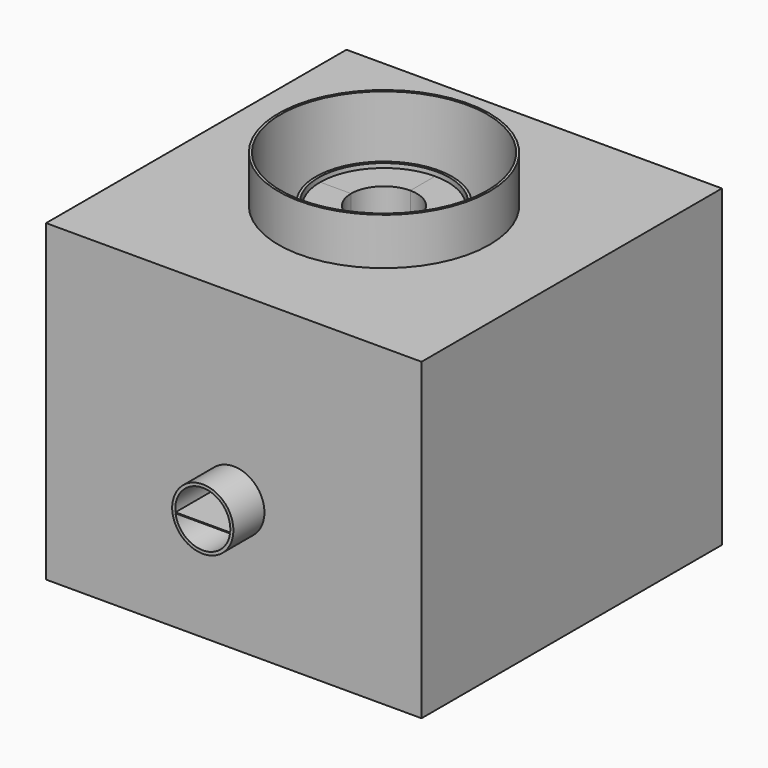
from build123d import *

# Parameters (mm, degrees)
F1_DEPTH       = 300
F0_W           = 400
F0_H           = 400
F0_R           = 112.5
F3_DEPTH       = 300
F0_R_2         = 110
F6_DEPTH       = 350
F2_W           = 400
F2_H           = 400
F7_DEPTH       = 10
F7_DEPTH_BACK  = 34.37157
F8_DEPTH       = 300
F9_R           = 72.7369791191
F9_R_2         = 69.9297965839
F10_DEPTH      = 293.61576
F4_R           = 30
F11_DEPTH      = 200.001
F12_R          = 32.6159593981
F12_R_2        = 29.3425223408
F13_DEPTH      = 41.30995
F13_DEPTH_BACK = 188.14221
F15_DEPTH      = 41.30995
F15_DEPTH_BACK = 187.07896
F16_R          = 35.0632832386
F17_DEPTH      = 410.93389


with BuildPart() as f1:
    # F0 (on Top) → F1 (new body)
    with BuildSketch(Plane.XY):
        with BuildLine():
            Line((0, 35), (0, 68))
            ThreePointArc((0, 68), (-48.0832611207, 48.0832611207), (-68, 0))
            Line((-68, 0), (-35, 0))
            ThreePointArc((-35, 0), (-24.7487373415, 24.7487373415), (0, 35))
        make_face()
    extrude(amount=F1_DEPTH)


with BuildPart() as f1b:
    # F0 (on Top) → F1, piece 2 (new body)
    with BuildSketch(Plane.XY):
        with BuildLine():
            ThreePointArc((0, -68), (48.0832611207, -48.0832611207), (68, 0))
            Line((68, 0), (35, 0))
            ThreePointArc((35, 0), (24.7487373415, -24.7487373415), (0, -35))
            Line((0, -35), (0, -68))
        make_face()
    extrude(amount=F1_DEPTH)


with BuildPart() as f3:
    # F0 (on Top) → F3 (new body)
    with BuildSketch(Plane.XY):
        Rectangle(F0_W, F0_H)
        Circle(F0_R, mode=Mode.SUBTRACT)
    extrude(amount=F3_DEPTH)

    # F2 (on Top) → F7 (join, two sides)
    with BuildSketch(Plane.XY) as f7_sk:
        Rectangle(F2_W, F2_H)
    extrude(amount=F7_DEPTH)
    extrude(f7_sk.sketch, amount=-F7_DEPTH_BACK)

    # F9 (on face) → F10 (join)
    with BuildSketch(Plane.XY.offset(10)):
        Circle(F9_R)
        Circle(F9_R_2, mode=Mode.SUBTRACT)
    extrude(amount=F10_DEPTH)


with BuildPart() as f6:
    # F0 (on Top) → F6 (new body)
    with BuildSketch(Plane.XY):
        Circle(F0_R)
        Circle(F0_R_2, mode=Mode.SUBTRACT)
    extrude(amount=F6_DEPTH)


with BuildPart() as f8:
    # F0 (on Top) → F8 (new body)
    with BuildSketch(Plane.XY):
        with BuildLine():
            ThreePointArc((-68, 0), (-48.0832611207, -48.0832611207), (0, -68))
            Line((0, -68), (0, -35))
            ThreePointArc((0, -35), (-24.7487373415, -24.7487373415), (-35, 0))
            Line((-35, 0), (-68, 0))
        make_face()
    extrude(amount=F8_DEPTH)


with BuildPart() as f8b:
    # F0 (on Top) → F8, piece 2 (new body)
    with BuildSketch(Plane.XY):
        with BuildLine():
            Line((35, 0), (68, 0))
            ThreePointArc((68, 0), (48.0832611207, 48.0832611207), (0, 68))
            Line((0, 68), (0, 35))
            ThreePointArc((0, 35), (24.7487373415, 24.7487373415), (35, 0))
        make_face()
    extrude(amount=F8_DEPTH)


with BuildPart() as f11_tool:
    # F4 (on Front) → F11 (new body, through all)
    with BuildSketch(Plane.XZ):
        with Locations((0, 104.252897203)):
            Circle(F4_R)
    extrude(amount=F11_DEPTH)


with BuildPart() as f1b_1:
    add(f1b.part)

    # F11: cut by f11_tool
    add(f11_tool.part, mode=Mode.SUBTRACT)


with BuildPart() as f3_1:
    add(f3.part)

    # F11: cut by f11_tool
    add(f11_tool.part, mode=Mode.SUBTRACT)


with BuildPart() as f6_1:
    add(f6.part)

    # F11: cut by f11_tool
    add(f11_tool.part, mode=Mode.SUBTRACT)


with BuildPart() as f8_1:
    add(f8.part)

    # F11: cut by f11_tool
    add(f11_tool.part, mode=Mode.SUBTRACT)


with BuildPart() as f13:
    # F12 (on face) → F13 (new body, two sides)
    with BuildSketch(Plane.XZ.offset(200)) as f13_sk:
        with Locations((0, 104.252897203)):
            Circle(F12_R)
        with Locations((0, 104.252897203)):
            Circle(F12_R_2, mode=Mode.SUBTRACT)
    extrude(amount=F13_DEPTH)
    extrude(f13_sk.sketch, amount=-F13_DEPTH_BACK)


with BuildPart() as f15:
    # F14 (on face) → F15 (new body, two sides)
    with BuildSketch(Plane.XZ.offset(200)) as f15_sk:
        Polygon((29.174895821, 101.1209535325), (-29.174895821, 101.1209535325), (-29.0519116779, 100.133425734), (29.0519116779, 100.133425734), align=None)
    extrude(amount=F15_DEPTH)
    extrude(f15_sk.sketch, amount=-F15_DEPTH_BACK)


with BuildPart() as f17_tool:
    # F16 (on face) → F17 (new body)
    with BuildSketch(Plane.XY.offset(10)):
        Circle(F16_R)
    extrude(amount=F17_DEPTH)


with BuildPart() as f1_1:
    add(f1.part)

    # F17: cut by f17_tool
    add(f17_tool.part, mode=Mode.SUBTRACT)


with BuildPart() as f1b_2:
    add(f1b_1.part)

    # F17: cut by f17_tool
    add(f17_tool.part, mode=Mode.SUBTRACT)


with BuildPart() as f8_2:
    add(f8_1.part)

    # F17: cut by f17_tool
    add(f17_tool.part, mode=Mode.SUBTRACT)


with BuildPart() as f8b_1:
    add(f8b.part)

    # F17: cut by f17_tool
    add(f17_tool.part, mode=Mode.SUBTRACT)


with BuildPart() as f13_1:
    add(f13.part)

    # F17: cut by f17_tool
    add(f17_tool.part, mode=Mode.SUBTRACT)


with BuildPart() as f15_1:
    add(f15.part)

    # F17: cut by f17_tool
    add(f17_tool.part, mode=Mode.SUBTRACT)


solid = Compound([f3_1.part, f6_1.part, f1_1.part, f1b_2.part, f8_2.part, f8b_1.part, f13_1.part, f15_1.part])
